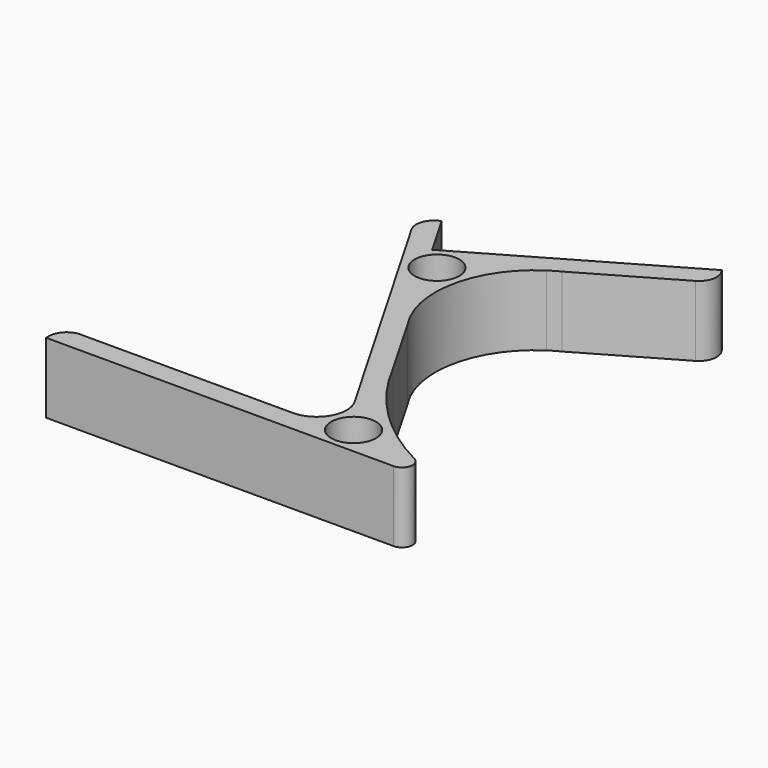
from build123d import *

# Parameters (mm, degrees)
F1_DEPTH = 20
F2_R     = 5
F3_R     = 6.35
F4_DEPTH = 25
F5_R     = 3


# Not quite as in the source:
# - a feature names something its author has since deleted; it is built from what else it names


with BuildPart() as f1:
    # F0 (on Top) → F1 (new body)
    with BuildSketch(Plane.XY):
        with BuildLine():
            Line((-90.3923048454, -24.3281582892), (-90.392, -30.3281582892))
            Line((-90.392, -30.3281582892), (0, -30.3281582892))
            Line((0, -30.3281582892), (25, -30.3281582892))
            ThreePointArc((25, -30.3281582892), (-1.9589555892, -17.2068745453), (-20.9641016151, 5.9827308433))
            Line((-20.9641016151, 5.9827308433), (-31.9301010618, 24.9763990407))
            ThreePointArc((-31.9301010618, 24.9763990407), (-36.0778921244, 46.2412468008), (-23.9743052597, 64.2106960401))
            ThreePointArc((-23.9743052597, 64.2106960401), (-22.4887853878, 65.1306303747), (-20.9493389483, 65.9571611543))
            Line((-20.9493389483, 65.9571611543), (9.3615501841, 83.4571611543))
            Line((9.3615501841, 83.4571611543), (6.3615501841, 88.653313577))
            Line((6.3615501841, 88.653313577), (-49.9301010618, 56.153313577))
            Line((-49.9301010618, 56.153313577), (-56.9301010618, 68.2776692299))
            Line((-56.9301010618, 68.2776692299), (-62.1262534846, 65.2776692299))
            Line((-62.1262534846, 65.2776692299), (-53.6935750346, 50.6718417108))
            Line((-53.6935750346, 50.6718417108), (-17.8923048454, -11.3377772324))
            ThreePointArc((-17.8923048454, -11.3377772324), (-17.7483786227, -11.5778506661), (-17.6124320417, -11.8225311482))
            Line((-17.6124320417, -11.8225311482), (-10.3923048454, -24.3281582892))
            Line((-10.3923048454, -24.3281582892), (-24.8325592379, -24.3281582892))
            ThreePointArc((-24.8325592379, -24.3281582892), (-25.1124320417, -24.3327653375), (-25.3923048454, -24.3281582892))
            Line((-25.3923048454, -24.3281582892), (-90.3923048454, -24.3281582892))
        make_face()
        with BuildLine():
            ThreePointArc((-17.6124320417, -11.8225311482), (-17.7483786227, -20.0811271137), (-24.8325592379, -24.3281582892))
            Line((-24.8325592379, -24.3281582892), (-10.3923048454, -24.3281582892))
            Line((-10.3923048454, -24.3281582892), (-17.6124320417, -11.8225311482))
        make_face()
    extrude(amount=F1_DEPTH)

    # F2
    f2_edges = [f1.edges().sort_by_distance(p)[0] for p in [
        (-90.392305, -24.328158, 10),
        (-62.126253, 65.277669, 10),
        (9.36155, 83.457161, 10),
    ]]
    fillet(f2_edges, radius=F2_R)

    # F3 (on face) → F4 (cut)
    with BuildSketch(Plane.XY.offset(20)):
        with Locations((-43.719941363, 50.0970014554)):
            Circle(F3_R)
        with Locations((-9.4799492508, -22.3026443273)):
            Circle(F3_R)
    extrude(amount=-F4_DEPTH, mode=Mode.SUBTRACT)

    # F5
    f5_edges = [f1.edges().sort_by_distance(p)[0] for p in [
        (25, -30.328158, 10),
    ]]
    fillet(f5_edges, radius=F5_R)


solid = f1.part
